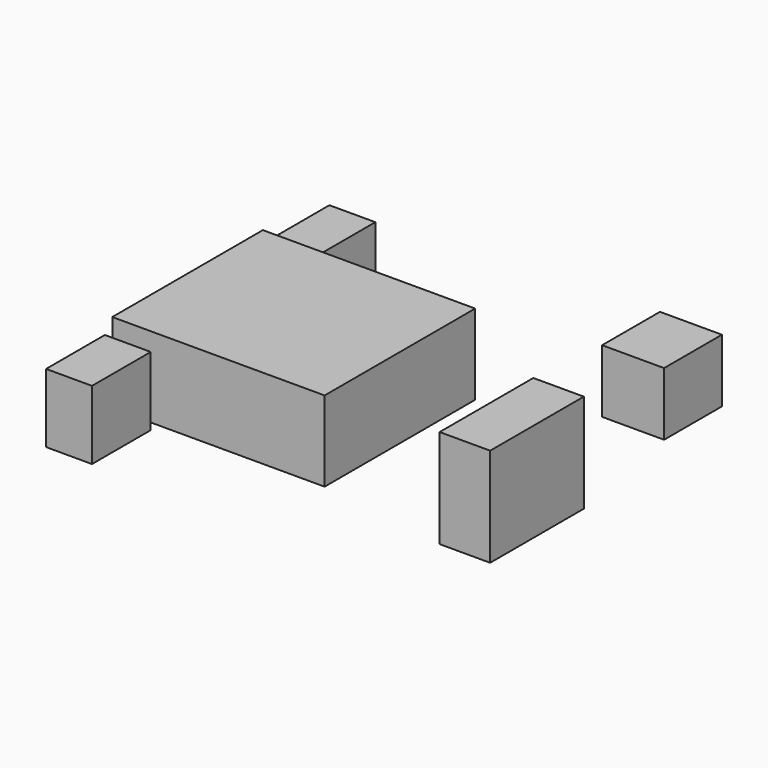
from build123d import *

# Parameters (mm, degrees)
F0_W     = 508
F0_H     = 812.8
F2_DEPTH = 762
F0_W_2   = 2349.5
F0_H_2   = 2082.8
F3_DEPTH = 889
F0_W_3   = 558.8
F0_H_3   = 1295.4
F5_DEPTH = 1092.2
F0_W_4   = 685.8
F0_H_4   = 800.1
F6_DEPTH = 698.5


# Not quite as in the source:
# - the program builds the solid bodies; features that only make, move or delete a surface that nothing else refers to are left out


with BuildPart() as f2:
    # F0 (on Top) → F2 (new body)
    with BuildSketch(Plane.XY):
        with Locations((-1916.6557788849, -1560.0854158401)):
            Rectangle(F0_W, F0_H)
    extrude(amount=F2_DEPTH)


with BuildPart() as f2b:
    # F0 (on Top) → F2, piece 2 (new body)
    with BuildSketch(Plane.XY):
        with Locations((-1918.6471700668, 1548.560500145)):
            Rectangle(F0_W, F0_H)
    extrude(amount=F2_DEPTH)


with BuildPart() as f3:
    # F0 (on Top) → F3 (new body)
    with BuildSketch(Plane.XY):
        with Locations((-1003.3, 0)):
            Rectangle(F0_W_2, F0_H_2)
    extrude(amount=F3_DEPTH)


with BuildPart() as f5:
    # F0 (on Top) → F5 (new body)
    with BuildSketch(Plane.XY):
        with Locations((1898.65, -612.1559739113)):
            Rectangle(F0_W_3, F0_H_3)
    extrude(amount=F5_DEPTH)


with BuildPart() as f6:
    # F0 (on Top) → F6 (new body)
    with BuildSketch(Plane.XY):
        with Locations((1570.7222600937, 1876.5427314758)):
            Rectangle(F0_W_4, F0_H_4)
    extrude(amount=F6_DEPTH)


solid = Compound([f2.part, f2b.part, f3.part, f5.part, f6.part])
